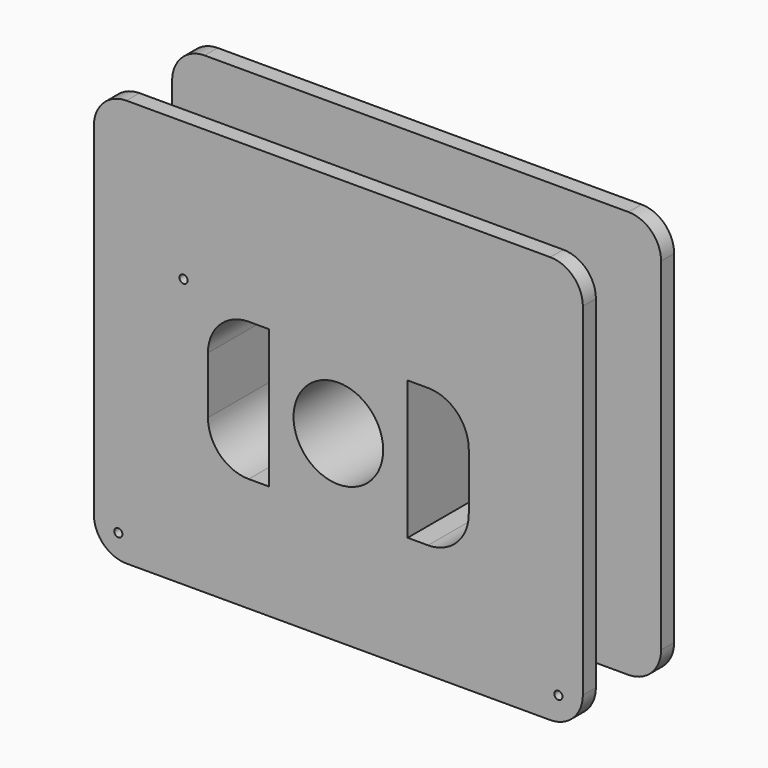
from build123d import *

# Parameters (mm, degrees)
F0_W      = 60
F0_H      = 50
F0_R      = 5.5
F1_DEPTH  = 2
F2_W      = 40
F2_H      = 25
F2_R      = 5.5
F3_DEPTH  = 10
F4_R      = 10
F5_W      = 60
F5_H      = 50
F5_R      = 5.5
F6_DEPTH  = 2
F7_R      = 4
F9_D      = 1
F9_DEPTH  = 3
F9_TIP    = 0.3004303095
F10_W     = 7.5
F10_H     = 17
F11_DEPTH = 25
F12_R     = 5


# Not quite as in the source:
# - a feature names something its author has since deleted; it is built from what else it names


with BuildPart() as f1:
    # F0 (on Front) → F1 (new body)
    with BuildSketch(Plane.XZ):
        with Locations((0, 2.5)):
            Rectangle(F0_W, F0_H)
        Circle(F0_R, mode=Mode.SUBTRACT)
    extrude(amount=F1_DEPTH)

    # F2 (on face) → F3 (join)
    with BuildSketch(Plane.XZ.offset(2)):
        Rectangle(F2_W, F2_H)
        Circle(F2_R, mode=Mode.SUBTRACT)
    extrude(amount=F3_DEPTH)

    # F4
    f4_edges = [f1.edges().sort_by_distance(p)[0] for p in [
        (20, -7, 12.5),
        (20, -7, -12.5),
        (-20, -7, -12.5),
        (-20, -7, 12.5),
    ]]
    fillet(f4_edges, radius=F4_R)

    # F5 (on face) → F6 (join)
    with BuildSketch(Plane.XZ.offset(12)):
        with Locations((0, 2.5)):
            Rectangle(F5_W, F5_H)
        Circle(F5_R, mode=Mode.SUBTRACT)
    extrude(amount=F6_DEPTH)

    # F7
    f7_edges = [f1.edges().sort_by_distance(p)[0] for p in [
        (30, -13, 27.5),
        (30, -1, 27.5),
        (30, -13, -22.5),
        (30, -1, -22.5),
        (-30, -13, -22.5),
        (-30, -1, -22.5),
        (-30, -13, 27.5),
        (-30, -1, 27.5),
    ]]
    fillet(f7_edges, radius=F7_R)

    # F9
    with Locations(Plane.XZ.offset(14)):
        with Locations((-19, 10.5), (-27, -19.5), (27, -19.5)):
            Hole(F9_D / 2, depth=F9_DEPTH)
            with Locations((0, 0, -(F9_DEPTH + F9_TIP / 2))):  # 118° drill point
                Cone(0, F9_D / 2, F9_TIP, mode=Mode.SUBTRACT)

    # F10 (on face) → F11 (cut)
    with BuildSketch(Plane.XZ.offset(14)):
        with Locations((-12.25, 0)):
            Rectangle(F10_W, F10_H)
        with Locations((12.25, 0)):
            Rectangle(F10_W, F10_H)
    extrude(amount=-F11_DEPTH, mode=Mode.SUBTRACT)

    # F12
    f12_edges = [f1.edges().sort_by_distance(p)[0] for p in [
        (16, -7, -8.5),
        (16, -7, 8.5),
        (-16, -7, 8.5),
        (-16, -7, -8.5),
    ]]
    fillet(f12_edges, radius=F12_R)


solid = f1.part
